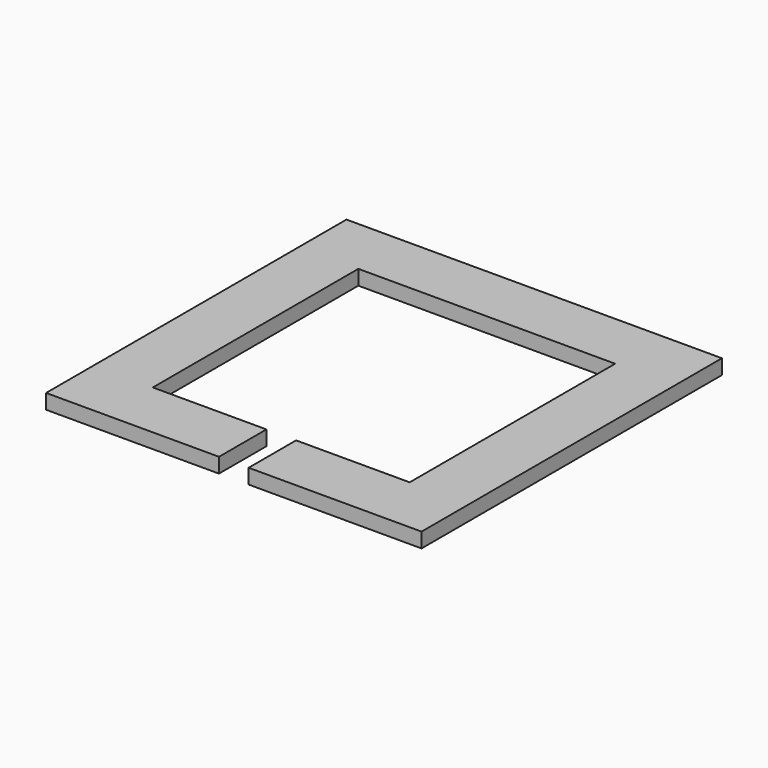
from build123d import *

# Parameters (mm, degrees)
F1_DEPTH = 3.175


# Not quite as in the source:
# - a length typed as a fraction of an inch, garbled in the dataset ("3 / 203.2 mm" for 3/8 in), is restored


with BuildPart() as f1:
    # F0 (on Top) → F1 (new body)
    with BuildSketch(Plane.XY):
        Polygon((40.2, 0), (-40.2, 0), (-40.2, -80.4), (-3.175, -80.4), (-3.175, -67.7), (-27.5, -67.7), (-27.5, -12.7), (27.5, -12.7), (27.5, -67.7), (3.175, -67.7), (3.175, -80.4), (40.2, -80.4), align=None)
    extrude(amount=F1_DEPTH)


solid = f1.part
